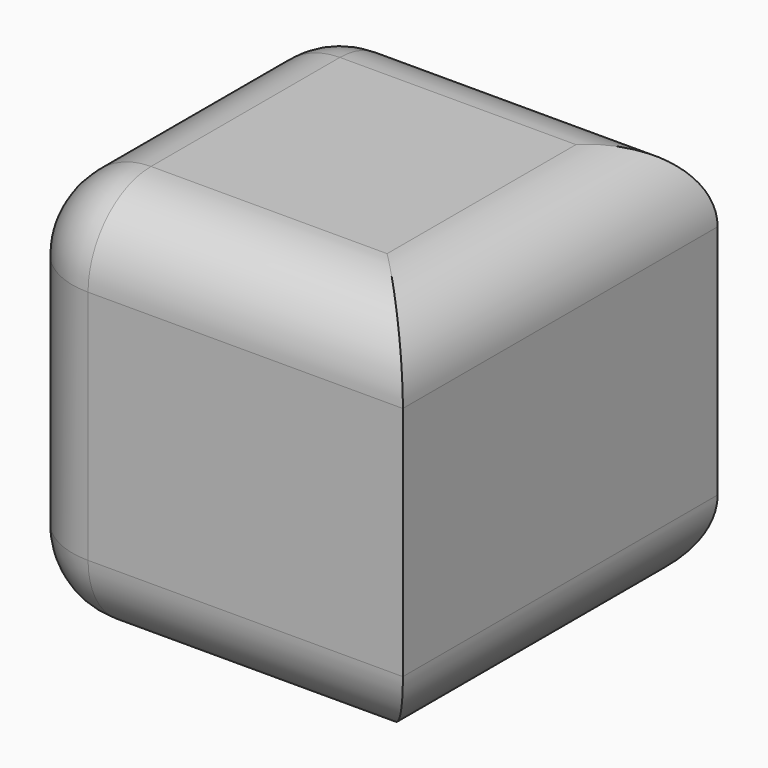
from build123d import *

# Parameters (mm, degrees)
F0_W     = 25
F0_H     = 25
F1_DEPTH = 25
F2_R     = 5
F3_T     = -3


# Not quite as in the source:
# - a shell that OpenCascade refuses in one call is made with other operations: the cavity is built on its own and cut out


with BuildPart() as f1:
    # F0 (on Front) → F1 (new body)
    with BuildSketch(Plane.XZ):
        with Locations((12.5, 12.5)):
            Rectangle(F0_W, F0_H)
    extrude(amount=F1_DEPTH)

    # F2
    f2_edges = [f1.edges().sort_by_distance(p)[0] for p in [
        (12.5, 0, 0),
        (25, -12.5, 0),
        (25, -12.5, 25),
        (12.5, 0, 25),
        (12.5, -25, 25),
        (0, -12.5, 25),
        (12.5, -25, 0),
        (0, -25, 12.5),
        (0, 0, 12.5),
        (0, -12.5, 0),
    ]]
    fillet(f2_edges, radius=F2_R)

    # F3: a shell. OpenCascade refuses it in one call, so the cavity is built on its own and cut out:
    # the body offset inwards by the wall thickness, plus a prism from it out through each open face.
    f3_core = offset(f1.part, amount=F3_T, mode=Mode.PRIVATE)
    f3_exits = [f3_core.faces().sort_by_distance(p)[0] for p in [
        (12.5, -12.5, 3),
    ]]
    add(f3_core, mode=Mode.SUBTRACT)
    extrude(f3_exits, amount=-F3_T, mode=Mode.SUBTRACT)


solid = f1.part
